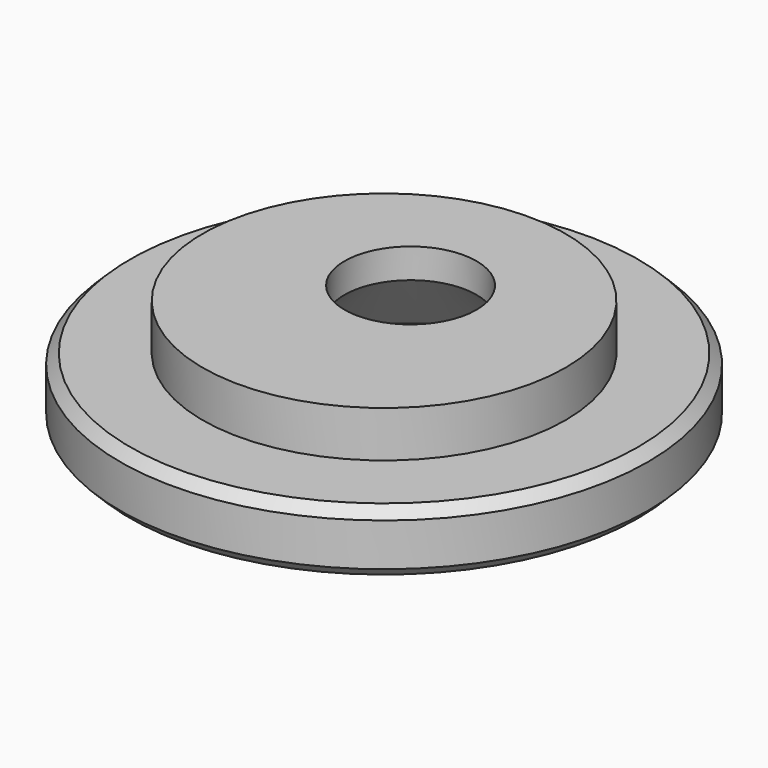
from build123d import *

# Parameters (mm, degrees)
F0_R     = 5.5
F0_R_2   = 2
F1_DEPTH = 3.3
F0_R_3   = 8
F2_DEPTH = 1.9
F3_SIZE  = 2.4
F4_SIZE  = 0.3


# Not quite as in the source:
# - a feature names something its author has since deleted; it is built from what else it names


with BuildPart() as f1:
    # F0 (on Top) → F1 (new body)
    with BuildSketch(Plane.XY):
        with Locations((0, -2)):
            Circle(F0_R)
        with Locations((0, -0.9976860601)):
            Circle(F0_R_2, mode=Mode.SUBTRACT)
    extrude(amount=F1_DEPTH)

    # F0 (on Top) → F2 (join)
    with BuildSketch(Plane.XY):
        with Locations((0, -2)):
            Circle(F0_R_3)
        with Locations((0, -2)):
            Circle(F0_R, mode=Mode.SUBTRACT)
    extrude(amount=F2_DEPTH)

    # F3
    f3_edges = [f1.edges().sort_by_distance(p)[0] for p in [
        (-2, -0.997686, 0),
    ]]
    chamfer(f3_edges, length=F3_SIZE)

    # F4
    f4_edges = [f1.edges().sort_by_distance(p)[0] for p in [
        (-8, -2, 1.9),
        (-8, -2, 0),
    ]]
    chamfer(f4_edges, length=F4_SIZE)


solid = f1.part
